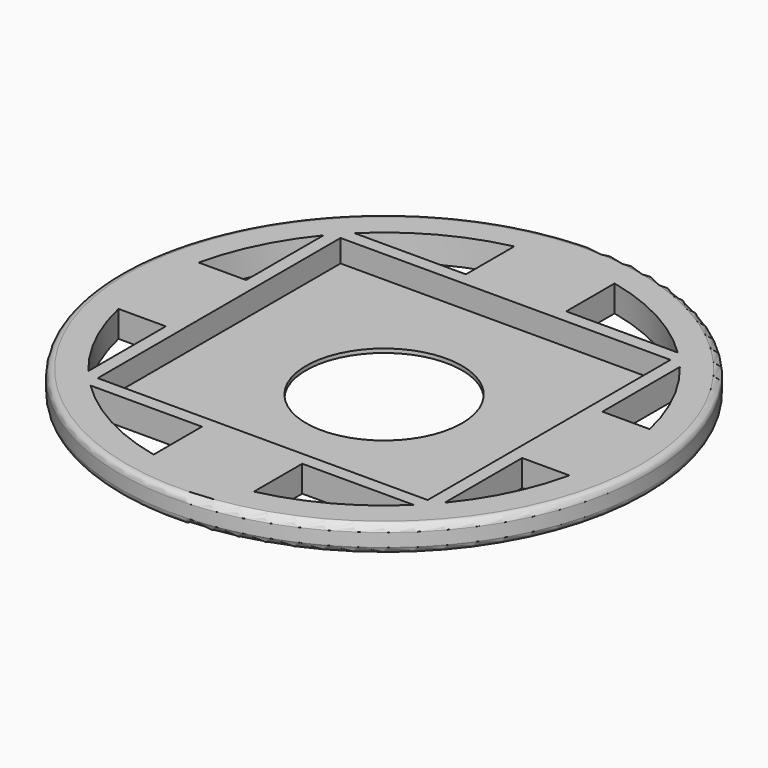
from build123d import *

# Parameters (mm, degrees)
F0_R     = 10
F1_DEPTH = 1
F2_W     = 12.5
F2_H     = 11.5
F3_DEPTH = 0.85
F5_R     = 2.9508175635
F6_DEPTH = 0.15
F7_R     = 0.25
F9_DEPTH = 1


# Not quite as in the source:
# - a feature names something its author has since deleted; it is built from what else it names


with BuildPart() as f1:
    # F0 (on Top) → F1 (new body)
    with BuildSketch(Plane.XY):
        Circle(F0_R)
    extrude(amount=F1_DEPTH)

    # F2 (on face) → F3 (cut)
    with BuildSketch(Plane.XY.offset(1)):
        with Locations((0, 0.0005259759)):
            Rectangle(F2_W, F2_H)
    extrude(amount=-F3_DEPTH, mode=Mode.SUBTRACT)

    # F5 (on offset) → F6 (cut)
    with BuildSketch(Plane.XY.offset(0.15)):
        Circle(F5_R)
    extrude(amount=-F6_DEPTH, mode=Mode.SUBTRACT)

    # F7
    f7_edges = [f1.edges().sort_by_distance(p)[0] for p in [
        (-10, 0, 1),
        (-10, 0, 0),
    ]]
    fillet(f7_edges, radius=F7_R)

    # F8 (on face) → F9 (cut, through all)
    with BuildSketch(Plane.XY.offset(1)):
        with BuildLine():
            Line((1.9, 8.5412235657), (1.9, 6.2505259759))
            Line((1.9, 6.2505259759), (6.1231874889, 6.2505259759))
            ThreePointArc((6.1231874889, 6.2505259759), (4.1718950409, 7.6914102587), (1.9, 8.5412235657))
        make_face()
        with BuildLine():
            Line((-6.75, 1.9), (-6.75, 5.5677643628))
            ThreePointArc((-6.75, 5.5677643628), (-7.8624743809, 3.8397912196), (-8.5412235657, 1.9))
            Line((-8.5412235657, 1.9), (-6.75, 1.9))
        make_face()
        with BuildLine():
            Line((-6.75, -5.5677643628), (-6.75, -1.9))
            Line((-6.75, -1.9), (-8.5412235657, -1.9))
            ThreePointArc((-8.5412235657, -1.9), (-7.8624743809, -3.8397912196), (-6.75, -5.5677643628))
        make_face()
        with BuildLine():
            Line((-1.9, -6.2505259759), (-6.1231874889, -6.2505259759))
            ThreePointArc((-6.1231874889, -6.2505259759), (-4.1718950409, -7.6914102587), (-1.9, -8.5412235657))
            Line((-1.9, -8.5412235657), (-1.9, -6.2505259759))
        make_face()
        with BuildLine():
            ThreePointArc((1.9, -8.5412235657), (4.1718950409, -7.6914102587), (6.1231874889, -6.2505259759))
            Line((6.1231874889, -6.2505259759), (1.9, -6.2505259759))
            Line((1.9, -6.2505259759), (1.9, -8.5412235657))
        make_face()
        with BuildLine():
            Line((8.5412235657, -1.9), (6.75, -1.9))
            Line((6.75, -1.9), (6.75, -5.5677643628))
            ThreePointArc((6.75, -5.5677643628), (7.8624743809, -3.8397912196), (8.5412235657, -1.9))
        make_face()
        with BuildLine():
            ThreePointArc((8.5412235657, 1.9), (7.8624743809, 3.8397912196), (6.75, 5.5677643628))
            Line((6.75, 5.5677643628), (6.75, 1.9))
            Line((6.75, 1.9), (8.5412235657, 1.9))
        make_face()
        with BuildLine():
            Line((-6.1231874889, 6.2505259759), (-1.9, 6.2505259759))
            Line((-1.9, 6.2505259759), (-1.9, 8.5412235657))
            ThreePointArc((-1.9, 8.5412235657), (-4.1718950409, 7.6914102587), (-6.1231874889, 6.2505259759))
        make_face()
    extrude(amount=-F9_DEPTH, mode=Mode.SUBTRACT)


solid = f1.part
